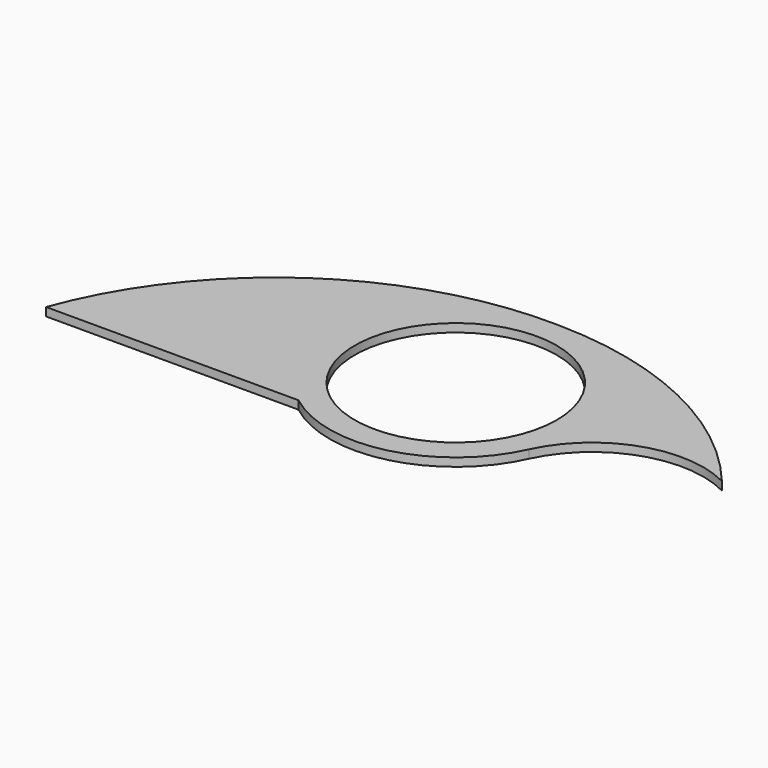
from build123d import *

# Parameters (mm, degrees)
F0_R     = 12.7
F1_DEPTH = 0.8382
F3_R     = 10.1600000635
F4_DEPTH = 18.288
F5_DEPTH = 0.8382
F7_DEPTH = 0.8382


# Not quite as in the source:
# - a feature of the source that left no trace in its solid (it failed there, or was rolled back) is left out


with BuildPart() as f1:
    # F0 (on Top) → F1 (new body)
    with BuildSketch(Plane.XY):
        Circle(F0_R)
    extrude(amount=F1_DEPTH)

    # F3 (on face) → F4 (cut)
    with BuildSketch(Plane.XY.offset(0.8382)):
        Circle(F3_R)
    extrude(amount=-F4_DEPTH, mode=Mode.SUBTRACT)

    # F2 (on face) → F5 (join)
    with BuildSketch(Plane.XY.offset(0.8382)):
        with BuildLine():
            Line((-33.1810780452, -10.0371721343), (-7.7810780452, -10.0371721343))
            ThreePointArc((-7.7810780452, -10.0371721343), (-12.0158663047, 4.1120502121), (0, 12.7))
            ThreePointArc((0, 12.7), (-20.2325604445, 6.6463315632), (-33.1810780452, -10.0371721343))
        make_face()
    extrude(amount=-F5_DEPTH)

    # F6 (on face) → F7 (join)
    with BuildSketch(Plane.XY.offset(0.8382)):
        with BuildLine():
            ThreePointArc((11.5657650484, -5.2462442609), (18.062719128, 0.5983562843), (26.7811901867, 0))
            ThreePointArc((26.7811901867, 0), (14.9176093432, 9.260079703), (0.265657769, 12.6972211901))
            ThreePointArc((0.265657769, 12.6972211901), (10.7465170902, 6.7677448556), (11.5657650484, -5.2462442609))
        make_face()
    extrude(amount=-F7_DEPTH)


solid = f1.part
